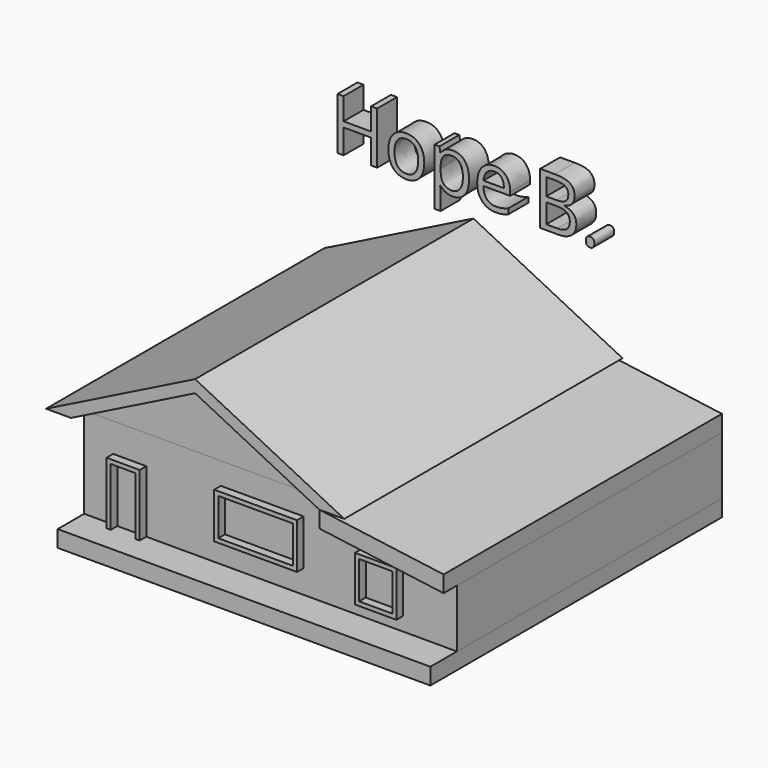
from build123d import *

# Parameters (mm, degrees)
F1_DEPTH     = 12801.6
F2_DEPTH     = 12192
F0_W         = 3048
F0_H         = 1676.4
F0_W_2       = 1524
F3_DEPTH     = 12192
F0_W_3       = 914.4
F0_H_2       = 2133.6
F4_DEPTH     = 12192
F0_W_4       = 2743.2
F0_H_3       = 1371.6
F0_W_5       = 1219.2
F0_W_6       = 4572
F0_H_4       = 609.6
F5_DEPTH     = 13411.2
F6_DEPTH     = 12496.8
F7_TEXT_SIZE = 2686.6217454274
F8_DEPTH     = 914.4
F9_W         = 1524
F9_H         = 1524
F10_DEPTH    = 152.4


# Not quite as in the source:
# - Text() gives the source's letters only with a copy of the font that has no kerning and outlines rounded to 1/6400 em; it was checked with that copy


with BuildPart() as f1:
    # F0 (on Front) → F1 (new body)
    with BuildSketch(Plane.XZ):
        Polygon((-5486.4, 0), (-4572, 0), (0, 2286), (0, 2743.2), align=None)
        Polygon((0, 2286), (4572, 0), (5486.4, 0), (0, 2743.2), align=None)
    extrude(amount=F1_DEPTH)



with BuildPart() as f1b:
    # F0 (on Front) → F1, piece 2 (new body)
    with BuildSketch(Plane.XZ):
        Polygon((9144, -609.6), (4572, 0), (4572, -609.6), (9144, -1219.2), align=None)
    extrude(amount=F1_DEPTH)


with BuildPart() as f1_1:
    add(f1.part)

    add(f1b.part)  # F2 merges F1b
    # F0 (on Front) → F2 (join)
    with BuildSketch(Plane.XZ):
        Polygon((-4572, 0), (0, 0), (0, 2286), align=None)
        Polygon((0, 2286), (0, 0), (4572, 0), align=None)
    extrude(amount=F2_DEPTH)


with BuildPart() as f3:
    # F0 (on Front) → F3 (new body)
    with BuildSketch(Plane.XZ):
        Polygon((4572, 0), (0, 0), (-4572, 0), (-4572, -3352.8), (-3505.2000017166, -3352.8), (-3505.2000017166, -1066.7999982834), (-2285.9999982834, -1066.7999982834), (-2285.9999982834, -3352.8), (4572, -3352.8), (4572, -609.6), align=None)
        with Locations((1981.2, -1650.7688323975)):
            Rectangle(F0_W, F0_H, mode=Mode.SUBTRACT)
        Polygon((9144, -1219.2), (4572, -609.6), (4572, -3352.8), (9144, -3352.8), align=None)
        with Locations((6400.8, -2011.185244751)):
            Rectangle(F0_W_2, F0_H, mode=Mode.SUBTRACT)
    extrude(amount=F3_DEPTH)

    # F9 (on face) → F10 (join)
    with BuildSketch(Plane(origin=(-4572, 0, 0), x_dir=(0, -1, 0), z_dir=(-1, 0, 0))):
        with Locations((2919.5521717072, -1533.3658103943)):
            Rectangle(F9_W, F9_H)
        with Locations((9231.4816360474, -1680.302942276)):
            Rectangle(F9_W, F9_H)
    extrude(amount=F10_DEPTH)


with BuildPart() as f4:
    # F0 (on Front) → F4 (new body)
    with BuildSketch(Plane.XZ):
        with Locations((-2895.6, -2286)):
            Rectangle(F0_W_3, F0_H_2)
    extrude(amount=F4_DEPTH)


with BuildPart() as f4b:
    # F0 (on Front) → F4, piece 2 (new body)
    with BuildSketch(Plane.XZ):
        with Locations((1981.2, -1650.7688323975)):
            Rectangle(F0_W_4, F0_H_3)
    extrude(amount=F4_DEPTH)


with BuildPart() as f4c:
    # F0 (on Front) → F4, piece 3 (new body)
    with BuildSketch(Plane.XZ):
        with Locations((6400.8, -2011.185244751)):
            Rectangle(F0_W_5, F0_H_3)
    extrude(amount=F4_DEPTH)


with BuildPart() as f5:
    # F0 (on Front) → F5 (new body)
    with BuildSketch(Plane.XZ):
        Polygon((-3505.2000017166, -3352.8), (-4572, -3352.8), (-4572, -3962.4), (4572, -3962.4), (4572, -3352.8), (-2285.9999982834, -3352.8), (-2438.4, -3352.8), (-3352.8, -3352.8), align=None)
        with Locations((6858, -3657.6)):
            Rectangle(F0_W_6, F0_H_4)
    extrude(amount=F5_DEPTH)


with BuildPart() as f6:
    # F0 (on Front) → F6 (new body)
    with BuildSketch(Plane.XZ):
        Polygon((-3505.2000017166, -1066.7999982834), (-3505.2000017166, -3352.8), (-3352.8, -3352.8), (-3352.8, -1219.2), (-2438.4, -1219.2), (-2438.4, -3352.8), (-2285.9999982834, -3352.8), (-2285.9999982834, -1066.7999982834), align=None)
    extrude(amount=F6_DEPTH)


with BuildPart() as f6b:
    # F0 (on Front) → F6, piece 2 (new body)
    with BuildSketch(Plane.XZ):
        with Locations((1981.2, -1650.7688323975)):
            Rectangle(F0_W, F0_H)
        with Locations((1981.2, -1650.7688323975)):
            Rectangle(F0_W_4, F0_H_3, mode=Mode.SUBTRACT)
    extrude(amount=F6_DEPTH)


with BuildPart() as f6c:
    # F0 (on Front) → F6, piece 3 (new body)
    with BuildSketch(Plane.XZ):
        with Locations((6400.8, -2011.185244751)):
            Rectangle(F0_W_2, F0_H)
        with Locations((6400.8, -2011.185244751)):
            Rectangle(F0_W_5, F0_H_3, mode=Mode.SUBTRACT)
    extrude(amount=F6_DEPTH)


with BuildPart() as f8:
    # F7 (on Front) → F8 (new body)
    with BuildSketch(Plane.XZ):
        with Locations((-4532.5155258179, 3845.4265594482)):
            Text('Hope B.', F7_TEXT_SIZE, font='Open Sans', text_align=(TextAlign.LEFT, TextAlign.BOTTOM))
    extrude(amount=F8_DEPTH)


solid = Compound([f1_1.part, f3.part, f4.part, f4b.part, f4c.part, f5.part, f6.part, f6b.part, f6c.part, f8.part])
